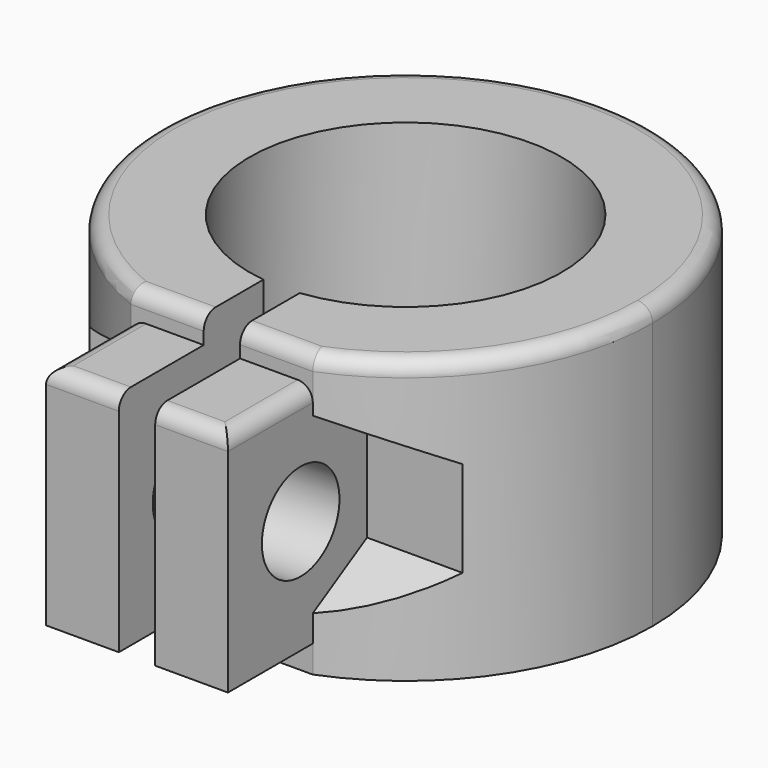
from build123d import *

# Parameters (mm, degrees)
F0_R      = 5.15
F1_DEPTH  = 9.3
F2_W      = 1.2
F2_H      = 13.8570601121
F3_DEPTH  = 9.301
F4_W      = 3.5
F4_H      = 0.9
F5_DEPTH  = 25
F7_R      = 1.6
F8_DEPTH  = 21.151
F10_DEPTH = 25
F12_DEPTH = 25
F13_R     = 0.5


with BuildPart() as f1:
    # F0 (on Top) → F1 (new body)
    with BuildSketch(Plane.XY):
        with BuildLine():
            ThreePointArc((3, -7.5777635223), (6.7406416609, -4.5810752013), (8.15, 0))
            ThreePointArc((8.15, 0), (-4.5810752013, 6.7406416609), (-3, -7.5777635223))
            Line((-3, -7.5777635223), (3, -7.5777635223))
        make_face()
        Circle(F0_R, mode=Mode.SUBTRACT)
        with BuildLine():
            Line((3, -7.5777635223), (-3, -7.5777635223))
            ThreePointArc((-3, -7.5777635223), (0, -8.15), (3, -7.5777635223))
        make_face()
        with BuildLine():
            ThreePointArc((3, -7.5777635223), (0, -8.15), (-3, -7.5777635223))
            Line((-3, -7.5777635223), (-3, -11.0777635223))
            Line((-3, -11.0777635223), (3, -11.0777635223))
            Line((3, -11.0777635223), (3, -7.5777635223))
        make_face()
    extrude(amount=F1_DEPTH)

    # F2 (on Top) → F3 (cut, through all)
    with BuildSketch(Plane.XY):
        with Locations((0, -6.928530056)):
            Rectangle(F2_W, F2_H)
    extrude(amount=F3_DEPTH, mode=Mode.SUBTRACT)

    # F4 (on face) → F5 (cut)
    with BuildSketch(Plane(origin=(-3, 0, 0), x_dir=(0, -1, 0), z_dir=(-1, 0, 0))):
        with Locations((9.3277635223, 8.85)):
            Rectangle(F4_W, F4_H)
        with Locations((9.3277635223, 0.45)):
            Rectangle(F4_W, F4_H)
    extrude(amount=-F5_DEPTH, mode=Mode.SUBTRACT)

    # F7 (on offset) → F8 (cut, through all)
    with BuildSketch(Plane(origin=(-13, 0, 0), x_dir=(0, -1, 0), z_dir=(-1, 0, 0))):
        with Locations((8.0777635223, 4.65)):
            Circle(F7_R)
    extrude(amount=-F8_DEPTH, mode=Mode.SUBTRACT)

    # F9 (on face) → F10 (cut)
    with BuildSketch(Plane(origin=(-3, 0, 0), x_dir=(0, -1, 0), z_dir=(-1, 0, 0))):
        Polygon((10.8127635223, 6.2290529862), (8.0777635223, 7.8081059725), (5.3427635223, 6.2290529862), (5.3427635223, 3.0709470138), (8.0777635223, 1.4918940275), (10.8127635223, 3.0709470138), align=None)
    extrude(amount=F10_DEPTH, mode=Mode.SUBTRACT)

    # F11 (on face) → F12 (cut)
    with BuildSketch(Plane.YZ.offset(3)):
        Polygon((-5.3427635223, 3.0709470138), (-5.3427635223, 6.2290529862), (-8.0777635223, 7.8081059725), (-10.8127635223, 6.2290529862), (-10.8127635223, 3.0709470138), (-8.0777635223, 1.4918940275), align=None)
    extrude(amount=F12_DEPTH, mode=Mode.SUBTRACT)

    # F13
    f13_edges = [f1.edges().sort_by_distance(p)[0] for p in [
        (0, 8.15, 9.3),
        (3, -9.327764, 8.4),
        (-3, -9.327764, 8.4),
        (-1.8, -7.577764, 9.3),
        (1.8, -7.577764, 9.3),
        (1.8, -11.077764, 8.4),
        (-1.8, -11.077764, 8.4),
    ]]
    fillet(f13_edges, radius=F13_R)


solid = f1.part
